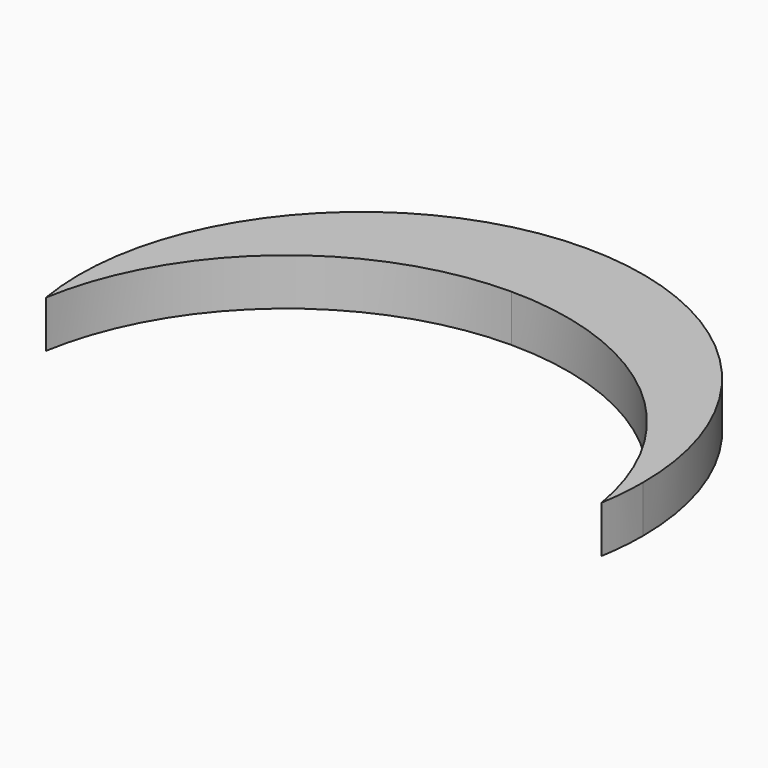
from build123d import *

# Parameters (mm, degrees)
F1_DEPTH = 6.35


with BuildPart() as f1:
    # F0 (on Top) → F1 (new body)
    with BuildSketch(Plane.XY):
        with BuildLine():
            ThreePointArc((37.5671066227, -6.35), (37.9665429182, -3.1861605167), (38.1, 0))
            ThreePointArc((38.1, 0), (26.9407683632, 26.9407683632), (0, 38.1))
            Line((0, 38.1), (0, 25.4))
            ThreePointArc((0, 25.4), (24.5934442484, 16.399355663), (37.5671066227, -6.35))
        make_face()
        with BuildLine():
            Line((0, 25.4), (0, 38.1))
            ThreePointArc((0, 38.1), (-29.099355663, 24.5934442484), (-37.5671066227, -6.35))
            ThreePointArc((-37.5671066227, -6.35), (-24.5934442484, 16.399355663), (0, 25.4))
        make_face()
    extrude(amount=-F1_DEPTH)


solid = f1.part
